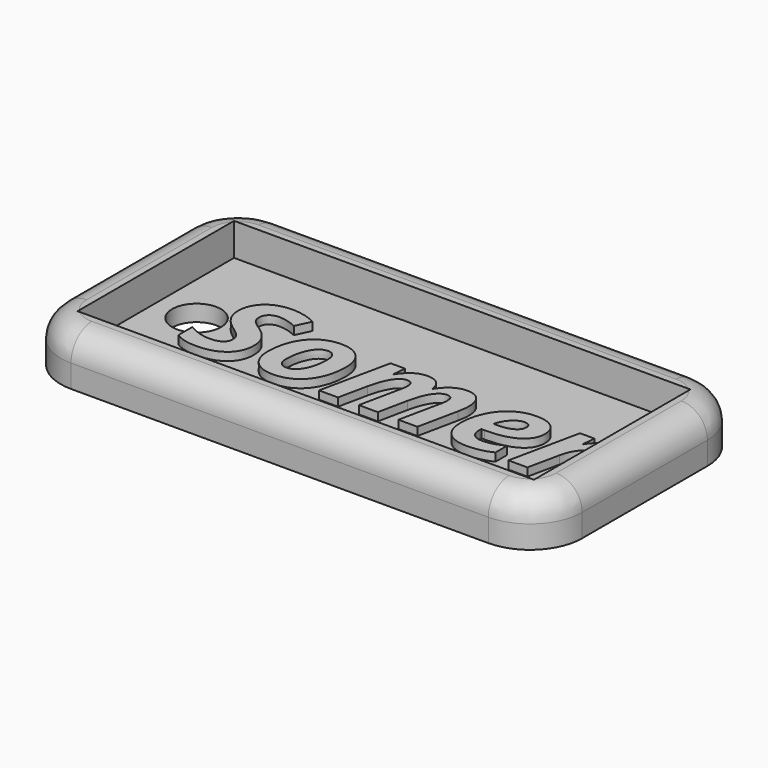
from build123d import *

# Parameters (mm, degrees)
F0_W         = 50.8
F0_H         = 25.4
F0_W_2       = 44.45
F0_H_2       = 19.05
F0_R         = 2.38125
F1_DEPTH     = 1.5875
F2_DEPTH     = 4.7625
F3_R         = 5.08
F4_T1_DEPTH  = 40.64
F4_T3_DEPTH  = 15.24
F4_T6_ANGLE  = 90
F4_T8_ANGLE  = 90
F4_T10_ANGLE = 90
F4_T12_ANGLE = 90
F5_TEXT_SIZE = 12.6193366267
F6_DEPTH     = 0.79375


# Not quite as in the source:
# - a fillet or chamfer that OpenCascade refuses, or shapes differently, is made with other operations: its cross-section is extruded or revolved along the edge and cut away or added
# - Text() gives the source's letters only with a copy of the font that has no kerning and outlines rounded to 1/6400 em; it was checked with that copy


with BuildPart() as f1:
    # F0 (on Top) → F1 (new body)
    with BuildSketch(Plane.XY):
        with Locations((25.4, 12.7)):
            Rectangle(F0_W, F0_H)
        with Locations((25.4, 12.7)):
            Rectangle(F0_W_2, F0_H_2, mode=Mode.SUBTRACT)
        with Locations((25.4, 12.7)):
            Rectangle(F0_W_2, F0_H_2)
        with Locations((7.14375, 12.7)):
            Circle(F0_R, mode=Mode.SUBTRACT)
    extrude(amount=F1_DEPTH)

    # F0 (on Top) → F2 (join)
    with BuildSketch(Plane.XY):
        with Locations((25.4, 12.7)):
            Rectangle(F0_W, F0_H)
        with Locations((25.4, 12.7)):
            Rectangle(F0_W_2, F0_H_2, mode=Mode.SUBTRACT)
    extrude(amount=F2_DEPTH)

    # F3
    f3_edges = [f1.edges().sort_by_distance(p)[0] for p in [
        (50.8, 0, 2.38125),
        (0, 0, 2.38125),
        (50.8, 25.4, 2.38125),
        (0, 25.4, 2.38125),
    ]]
    fillet(f3_edges, radius=F3_R)

    # F4: fillet of radius 2.54 on 8 edges, made by hand

    # F4_s2 → F4_t1 (cut)
    with BuildSketch(Plane.YZ.offset(5.08)):
        with BuildLine():
            ThreePointArc((2.54, 4.7625), (0.7439487758, 4.0185512242), (0, 2.2225))
            Line((0, 2.2225), (0, 4.7625))
            Line((0, 4.7625), (2.54, 4.7625))
        make_face()
        with BuildLine():
            ThreePointArc((22.86, 4.7625), (24.6560512242, 4.0185512242), (25.4, 2.2225))
            Line((25.4, 2.2225), (25.4, 4.7625))
            Line((25.4, 4.7625), (22.86, 4.7625))
        make_face()
    extrude(amount=F4_T1_DEPTH, mode=Mode.SUBTRACT)

    # F4_s4 → F4_t3 (cut)
    with BuildSketch(Plane.XZ.offset(-20.32)):
        with BuildLine():
            ThreePointArc((48.26, 4.7625), (50.0560512242, 4.0185512242), (50.8, 2.2225))
            Line((50.8, 2.2225), (50.8, 4.7625))
            Line((50.8, 4.7625), (48.26, 4.7625))
        make_face()
        with BuildLine():
            ThreePointArc((0, 2.2225), (0.7439487758, 4.0185512242), (2.54, 4.7625))
            Line((2.54, 4.7625), (0, 4.7625))
            Line((0, 4.7625), (0, 2.2225))
        make_face()
    extrude(amount=F4_T3_DEPTH, mode=Mode.SUBTRACT)

    # F4_s5 → F4_t6 (revolve, cut)
    with BuildSketch(Plane.XZ.offset(-20.32)):
        with BuildLine():
            ThreePointArc((2.54, 4.7625), (0.7439487758, 4.0185512242), (0, 2.2225))
            Line((0, 2.2225), (0, 4.7625))
            Line((0, 4.7625), (2.54, 4.7625))
        make_face()
    revolve(axis=Axis((5.08, 20.32, 4.7625), (0, 0, -1)), revolution_arc=F4_T6_ANGLE, mode=Mode.SUBTRACT)

    # F4_s7 → F4_t8 (revolve, cut)
    with BuildSketch(Plane.XZ.offset(-5.08)):
        with BuildLine():
            ThreePointArc((2.54, 4.7625), (0.7439487758, 4.0185512242), (0, 2.2225))
            Line((0, 2.2225), (0, 4.7625))
            Line((0, 4.7625), (2.54, 4.7625))
        make_face()
    revolve(axis=Axis((5.08, 5.08, 4.7625), (0, 0, 1)), revolution_arc=F4_T8_ANGLE, mode=Mode.SUBTRACT)

    # F4_s9 → F4_t10 (revolve, cut)
    with BuildSketch(Plane.XZ.offset(-20.32)):
        with BuildLine():
            ThreePointArc((48.26, 4.7625), (50.0560512242, 4.0185512242), (50.8, 2.2225))
            Line((50.8, 2.2225), (50.8, 4.7625))
            Line((50.8, 4.7625), (48.26, 4.7625))
        make_face()
    revolve(axis=Axis((45.72, 20.32, 4.7625), (0, 0, 1)), revolution_arc=F4_T10_ANGLE, mode=Mode.SUBTRACT)

    # F4_s11 → F4_t12 (revolve, cut)
    with BuildSketch(Plane.XZ.offset(-5.08)):
        with BuildLine():
            ThreePointArc((48.26, 4.7625), (50.0560512242, 4.0185512242), (50.8, 2.2225))
            Line((50.8, 2.2225), (50.8, 4.7625))
            Line((50.8, 4.7625), (48.26, 4.7625))
        make_face()
    revolve(axis=Axis((45.72, 5.08, 4.7625), (0, 0, -1)), revolution_arc=F4_T12_ANGLE, mode=Mode.SUBTRACT)

    # F5 (on face) → F6 (join)
    with BuildSketch(Plane.XY.offset(1.5875)):
        with Locations((8.509, 8.0252255486)):
            Text('Somer', F5_TEXT_SIZE, font='Open Sans', font_style=FontStyle.BOLDITALIC, text_align=(TextAlign.LEFT, TextAlign.BOTTOM))
    extrude(amount=F6_DEPTH)


solid = f1.part
